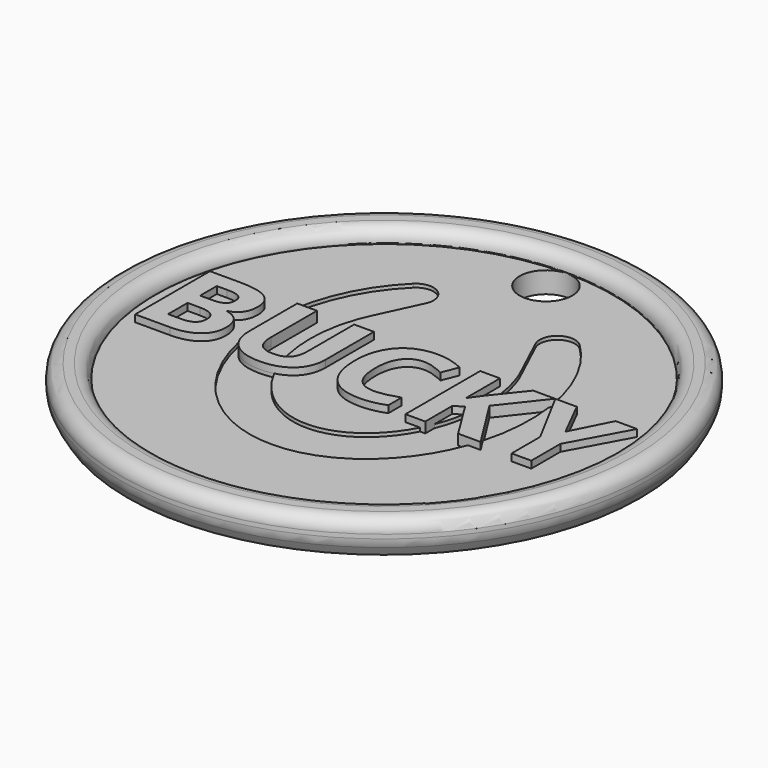
from build123d import *

# Parameters (mm, degrees)
F0_R          = 15
F1_DEPTH      = 2
F2_R          = 13
F3_DEPTH      = 0.8
F5_DEPTH      = 0.2
F7_TEXT_SIZE  = 7.4375467152
F8_DEPTH      = 0.4
F8_DEPTH_BACK = 0.5
F9_R          = 1.5
F10_DEPTH     = 2.001
F11_R         = 0.75
F12_SIZE2     = 0.4330127019
F12_SIZE      = 0.75
F13_R         = 1


# Not quite as in the source:
# - Text() gives the source's letters only with a copy of the font that has no kerning and outlines rounded to 1/6400 em; it was checked with that copy


with BuildPart() as f1:
    # F0 (on Top) → F1 (new body)
    with BuildSketch(Plane.XY):
        Circle(F0_R)
    extrude(amount=F1_DEPTH)

    # F2 (on face) → F3 (cut)
    with BuildSketch(Plane.XY.offset(2)):
        Circle(F2_R)
    extrude(amount=-F3_DEPTH, mode=Mode.SUBTRACT)

    # F4 (on face) → F5 (cut)
    with BuildSketch(Plane.XY.offset(1.2)):
        with BuildLine():
            add(Edge.make_bspline(
                [(-4.2132504423, 4.5), (-9.1287092918, -5.5), (0, -5.5), (9.1287092918, -5.5), (4.2132504423, 4.5)],
                knots=[4.1437786801, 4.1437786801, 4.1437786801, 6.2831853072, 6.2831853072, 8.4225919342, 8.4225919342, 8.4225919342], degree=2, weights=[1, 0.4803844614, 1, 0.4803844614, 1]))
            Line((-4.2132504423, 4.5), (-3.1141751045, 6.8569746681))
            ThreePointArc((-3.1141751045, 6.8569746681), (-3.4408457148, 8.0944676093), (-4.7170214144, 7.9971123276))
            add(Edge.make_bspline(
                [(-4.7170214144, 7.9971123276), (-21.1959928233, -8), (0, -8), (21.1959928233, -8), (4.7170214144, 7.9971123276)],
                knots=[3.8217767846, 3.8217767846, 3.8217767846, 6.2831853072, 6.2831853072, 8.7445938298, 8.7445938298, 8.7445938298], degree=2, weights=[1, 0.3335738859, 1, 0.3335738859, 1]))
            ThreePointArc((4.7170214144, 7.9971123276), (3.4408457148, 8.0944676093), (3.1141751045, 6.8569746681))
            Line((3.1141751045, 6.8569746681), (4.2132504423, 4.5))
        make_face()
    extrude(amount=-F5_DEPTH, mode=Mode.SUBTRACT)

    # F7 (on face) → F8 (join, two sides)
    with BuildSketch(Plane.XY.offset(1.2)) as f8_sk:
        with Locations((-12.7106511246, -2.6275168175)):
            Text('BUCKY', F7_TEXT_SIZE, font='Open Sans', font_style=FontStyle.BOLD, text_align=(TextAlign.LEFT, TextAlign.BOTTOM))
    extrude(amount=F8_DEPTH)
    extrude(f8_sk.sketch, amount=-F8_DEPTH_BACK)

    # F9 (on Top) → F10 (cut, through all)
    with BuildSketch(Plane.XY):
        with Locations((0, 11.5)):
            Circle(F9_R)
    extrude(amount=F10_DEPTH, mode=Mode.SUBTRACT)

    # F11
    f11_edges = [f1.edges().sort_by_distance(p)[0] for p in [
        (-15, 0, 2),
        (-13, 0, 2),
    ]]
    fillet(f11_edges, radius=F11_R)

    # F12
    f12_edges = [f1.edges().sort_by_distance(p)[0] for p in [
        (-15, 0, 0),
    ]]
    f12_side = f1.faces().sort_by_distance((-15, 0, 0.625))[0]
    chamfer(f12_edges, length=F12_SIZE, length2=F12_SIZE2, reference=f12_side)

    # F13
    f13_edges = [f1.edges().sort_by_distance(p)[0] for p in [
        (-15, 0, 0.75),
    ]]
    fillet(f13_edges, radius=F13_R)


solid = f1.part
